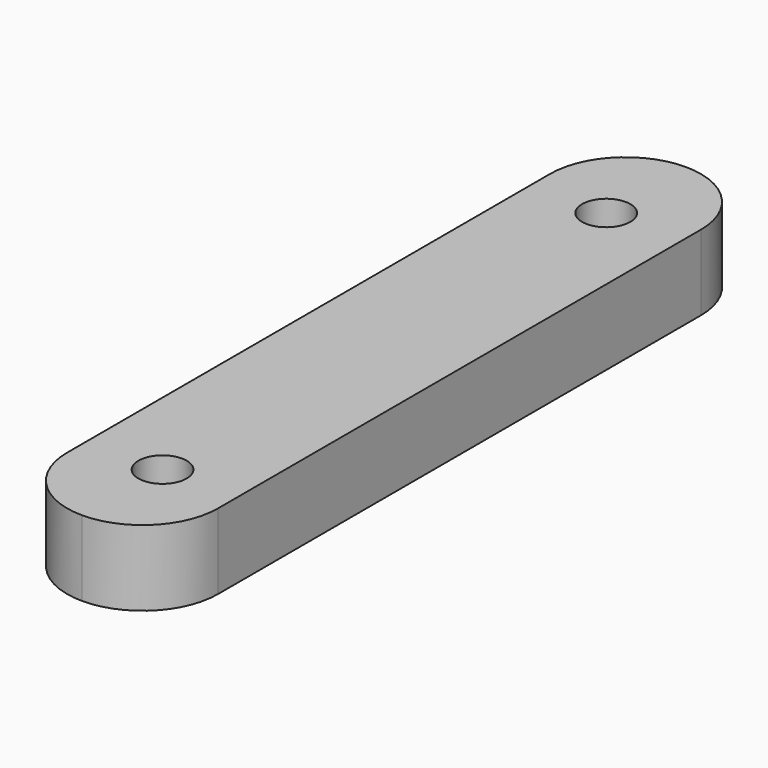
from build123d import *

# Parameters (mm, degrees)
F0_W     = 10
F0_H     = 50
F0_R     = 1.6
F1_DEPTH = 5
F2_R     = 4.99999


# Not quite as in the source:
# - a fillet or chamfer is up to 0.001 mm smaller than in the source, because OpenCascade refuses the exact size


with BuildPart() as f1:
    # F0 (on Top) → F1 (new body)
    with BuildSketch(Plane.XY):
        with Locations((-2.3096096679, -0.3726480128)):
            Rectangle(F0_W, F0_H)
        with Locations((-2.2665521668, -18.7726480128)):
            Circle(F0_R, mode=Mode.SUBTRACT)
        with Locations((-2.3018803907, 18.0273519872)):
            Circle(F0_R, mode=Mode.SUBTRACT)
    extrude(amount=F1_DEPTH)

    # F2 (radius 5 in the source; OpenCascade refuses exactly that, so slightly less here)
    f2_edges = [f1.edges().sort_by_distance(p)[0] for p in [
        (2.69039, -25.372648, 2.5),
        (-7.30961, -25.372648, 2.5),
        (2.69039, 24.627352, 2.5),
        (-7.30961, 24.627352, 2.5),
    ]]
    fillet(f2_edges, radius=F2_R)


solid = f1.part
